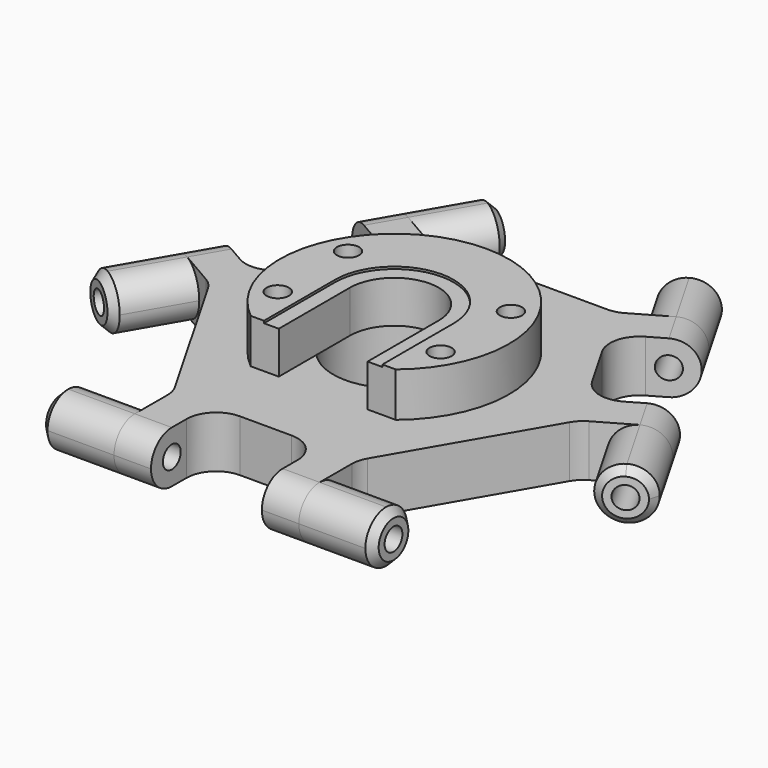
from build123d import *

# Parameters (mm, degrees)
F0_R      = 11
F0_R_2    = 8.25
F1_DEPTH  = 7
F2_W      = 5
F2_H      = 7
F3_DEPTH  = 10
F5_DEPTH  = 10
F6_R      = 1.5
F7_DEPTH  = 25
F8_SIZE   = 1
F10_DEPTH = 10
F11_R     = 1.5
F12_DEPTH = 25
F14_W     = 5
F14_H     = 7
F15_DEPTH = 10
F17_DEPTH = 10
F18_R     = 1.5
F19_DEPTH = 25
F20_SIZE  = 1
F22_DEPTH = 10
F23_R     = 1.5
F24_DEPTH = 25
F26_W     = 5
F26_H     = 7
F27_DEPTH = 10
F29_DEPTH = 10
F30_R     = 1.5
F31_DEPTH = 25
F32_SIZE  = 1
F34_DEPTH = 10
F35_R     = 1.5
F36_DEPTH = 25
F38_R     = 1.5
F39_DEPTH = 25
F40_R     = 3.4999
F41_R     = 4
F42_R     = 1.5
F43_DEPTH = 6
F45_DEPTH = 0.3
F46_R     = 10
F46_R_2   = 8.25
F47_DEPTH = 2


# Not quite as in the source:
# - a fillet or chamfer that OpenCascade refuses, or shapes differently, is made with other operations: its cross-section is extruded or revolved along the edge and cut away or added
# - a fillet or chamfer is up to 0.001 mm smaller than in the source, because OpenCascade refuses the exact size


with BuildPart() as f1:
    # F0 (on Top) → F1 (new body)
    with BuildSketch(Plane.XY):
        Polygon((24.999952403, -0.0487836684), (12.5422240976, 21.6262020402), (-12.4577283054, 21.6749857086), (-24.999952403, 0.0487836684), (-12.5422240976, -21.6262020402), (12.4577283054, -21.6749857086), align=None)
        Circle(F0_R, mode=Mode.SUBTRACT)
        Circle(F0_R)
        Circle(F0_R_2, mode=Mode.SUBTRACT)
    extrude(amount=F1_DEPTH)

    # F2 (on face) → F3 (join)
    with BuildSketch(Plane(origin=(-0.0422478961, -21.6505938744, 0), x_dir=(0.9999980961, -0.0019513467, 0), z_dir=(-0.0019513467, -0.9999980961, 0))):
        with Locations((-10, 3.5)):
            Rectangle(F2_W, F2_H)
        with Locations((10, 3.5)):
            Rectangle(F2_W, F2_H)
    extrude(amount=F3_DEPTH)

    # F4 (on face) → F5 (join)
    with BuildSketch(Plane(origin=(-12.4999762015, 0.0243918342, 0), x_dir=(-0.0019513467, -0.9999980961, 0), z_dir=(-0.9999980961, 0.0019513467, 0))):
        with BuildLine():
            ThreePointArc((28.1506350946, 0), (30.6255088288, 1.0251262658), (31.6506350946, 3.5))
            ThreePointArc((31.6506350946, 3.5), (30.6255088288, 5.9748737342), (28.1506350946, 7))
            ThreePointArc((28.1506350946, 7), (24.6506350946, 3.5), (28.1506350946, 0))
        make_face()
    extrude(amount=F5_DEPTH)

    # F6 (on face) → F7 (cut)
    with BuildSketch(Plane(origin=(-22.4999571627, 0.0439053016, 0), x_dir=(-0.0019513467, -0.9999980961, 0), z_dir=(-0.9999980961, 0.0019513467, 0))):
        with Locations((28.1506350946, 3.5)):
            Circle(F6_R)
    extrude(amount=-F7_DEPTH, mode=Mode.SUBTRACT)

    # F8
    f8_edges = [f1.edges().sort_by_distance(p)[0] for p in [
        (-22.554889, -28.106676, 7),
    ]]
    chamfer(f8_edges, length=F8_SIZE)

    # F9 (on face) → F10 (join)
    with BuildSketch(Plane(origin=(12.4999762015, -0.0243918342, 0), x_dir=(0.0019513467, 0.9999980961, 0), z_dir=(0.9999980961, -0.0019513467, 0))):
        with BuildLine():
            ThreePointArc((-28.1506350946, 0), (-25.6757613605, 1.0251262658), (-24.6506350946, 3.5))
            ThreePointArc((-24.6506350946, 3.5), (-25.6757613605, 5.9748737342), (-28.1506350946, 7))
            ThreePointArc((-28.1506350946, 7), (-30.6255088288, 5.9748737342), (-31.6506350946, 3.5))
            ThreePointArc((-31.6506350946, 3.5), (-30.6255088288, 1.0251262658), (-28.1506350946, 0))
        make_face()
    extrude(amount=F10_DEPTH)

    # F11 (on face) → F12 (cut)
    with BuildSketch(Plane(origin=(22.4999571627, -0.0439053016, 0), x_dir=(0.0019513467, 0.9999980961, 0), z_dir=(0.9999980961, -0.0019513467, 0))):
        with Locations((-28.1506350946, 3.5)):
            Circle(F11_R)
    extrude(amount=-F12_DEPTH, mode=Mode.SUBTRACT)

    # F13: chamfer of 1 on 1 edges, made by hand

    # F13_s1 → F13_t2 (revolve, cut)
    with BuildSketch(Plane.XY.offset(3.5)):
        Polygon((21.4381977031, -31.6925287905), (22.440147146, -30.6944820411), (22.4381957992, -31.6944801372), align=None)
    revolve(axis=Axis((22.4450255128, -28.1944868008, 3.5), (-0.9999980961, 0.0019513467, 0)), mode=Mode.SUBTRACT)

    # F14 (on face) → F15 (join)
    with BuildSketch(Plane(origin=(18.7710882503, 10.7887091859, 0), x_dir=(-0.4983091322, 0.8669994283, 0), z_dir=(0.8669994283, 0.4983091322, 0))):
        with Locations((-10, 3.5)):
            Rectangle(F14_W, F14_H)
        with Locations((10, 3.5)):
            Rectangle(F14_W, F14_H)
    extrude(amount=F15_DEPTH)

    # F16 (on face) → F17 (join)
    with BuildSketch(Plane(origin=(6.2288641527, -10.8374928543, 0), x_dir=(0.8669994283, 0.4983091322, 0), z_dir=(0.4983091322, -0.8669994283, 0))):
        with BuildLine():
            ThreePointArc((28.1506350946, 0), (30.6255088288, 1.0251262658), (31.6506350946, 3.5))
            ThreePointArc((31.6506350946, 3.5), (30.6255088288, 5.9748737342), (28.1506350946, 7))
            ThreePointArc((28.1506350946, 7), (24.6506350946, 3.5), (28.1506350946, 0))
        make_face()
    extrude(amount=F17_DEPTH)

    # F18 (on face) → F19 (cut)
    with BuildSketch(Plane(origin=(11.2119554749, -19.5074871378, 0), x_dir=(0.8669994283, 0.4983091322, 0), z_dir=(0.4983091322, -0.8669994283, 0))):
        with Locations((28.1506350946, 3.5)):
            Circle(F18_R)
    extrude(amount=-F19_DEPTH, mode=Mode.SUBTRACT)

    # F20
    f20_edges = [f1.edges().sort_by_distance(p)[0] for p in [
        (35.61854, -5.479769, 7),
    ]]
    chamfer(f20_edges, length=F20_SIZE)

    # F21 (on face) → F22 (join)
    with BuildSketch(Plane(origin=(-6.2288641527, 10.8374928543, 0), x_dir=(-0.8669994283, -0.4983091322, 0), z_dir=(-0.4983091322, 0.8669994283, 0))):
        with BuildLine():
            ThreePointArc((-28.1506350946, 0), (-25.6757613605, 1.0251262658), (-24.6506350946, 3.5))
            ThreePointArc((-24.6506350946, 3.5), (-25.6757613605, 5.9748737342), (-28.1506350946, 7))
            ThreePointArc((-28.1506350946, 7), (-30.6255088288, 5.9748737342), (-31.6506350946, 3.5))
            ThreePointArc((-31.6506350946, 3.5), (-30.6255088288, 1.0251262658), (-28.1506350946, 0))
        make_face()
    extrude(amount=F22_DEPTH)

    # F23 (on face) → F24 (cut)
    with BuildSketch(Plane(origin=(-11.2119554749, 19.5074871378, 0), x_dir=(-0.8669994283, -0.4983091322, 0), z_dir=(-0.4983091322, 0.8669994283, 0))):
        with Locations((-28.1506350946, 3.5)):
            Circle(F23_R)
    extrude(amount=-F24_DEPTH, mode=Mode.SUBTRACT)

    # F25: chamfer of 1 on 1 edges, made by hand

    # F25_s1 → F25_t2 (revolve, cut)
    with BuildSketch(Plane.XY.offset(3.5)):
        Polygon((16.7274361911, 34.4122882175), (15.3621276306, 34.7809785136), (16.2291270589, 35.2792876458), align=None)
    revolve(axis=Axis((13.1946290597, 33.5352056831, 3.5), (0.4983091322, -0.8669994283, 0)), mode=Mode.SUBTRACT)

    # F26 (on face) → F27 (join)
    with BuildSketch(Plane(origin=(-18.7288403542, 10.8618846885, 0), x_dir=(-0.5016889639, -0.8650480816, 0), z_dir=(-0.8650480816, 0.5016889639, 0))):
        with Locations((10, 3.5)):
            Rectangle(F26_W, F26_H)
        with Locations((-10, 3.5)):
            Rectangle(F26_W, F26_H)
    extrude(amount=F27_DEPTH)

    # F28 (on face) → F29 (join)
    with BuildSketch(Plane(origin=(6.2711120488, 10.8131010201, 0), x_dir=(-0.8650480816, 0.5016889639, 0), z_dir=(0.5016889639, 0.8650480816, 0))):
        with BuildLine():
            ThreePointArc((28.1506350946, 0), (30.6255088288, 1.0251262658), (31.6506350946, 3.5))
            ThreePointArc((31.6506350946, 3.5), (30.6255088288, 5.9748737342), (28.1506350946, 7))
            ThreePointArc((28.1506350946, 7), (24.6506350946, 3.5), (28.1506350946, 0))
        make_face()
    extrude(amount=F29_DEPTH)

    # F30 (on face) → F31 (cut)
    with BuildSketch(Plane(origin=(11.2880016879, 19.4635818362, 0), x_dir=(-0.8650480816, 0.5016889639, 0), z_dir=(0.5016889639, 0.8650480816, 0))):
        with Locations((28.1506350946, 3.5)):
            Circle(F30_R)
    extrude(amount=-F31_DEPTH, mode=Mode.SUBTRACT)

    # F32
    f32_edges = [f1.edges().sort_by_distance(p)[0] for p in [
        (-13.063651, 33.586445, 7),
    ]]
    chamfer(f32_edges, length=F32_SIZE)

    # F33 (on face) → F34 (join)
    with BuildSketch(Plane(origin=(-6.2711120488, -10.8131010201, 0), x_dir=(0.8650480816, -0.5016889639, 0), z_dir=(-0.5016889639, -0.8650480816, 0))):
        with BuildLine():
            ThreePointArc((-28.1506350946, 0), (-25.6757613605, 1.0251262658), (-24.6506350946, 3.5))
            ThreePointArc((-24.6506350946, 3.5), (-25.6757613605, 5.9748737342), (-28.1506350946, 7))
            ThreePointArc((-28.1506350946, 7), (-30.6255088288, 5.9748737342), (-31.6506350946, 3.5))
            ThreePointArc((-31.6506350946, 3.5), (-30.6255088288, 1.0251262658), (-28.1506350946, 0))
        make_face()
    extrude(amount=F34_DEPTH)

    # F35 (on face) → F36 (cut)
    with BuildSketch(Plane(origin=(-11.2880016879, -19.4635818362, 0), x_dir=(0.8650480816, -0.5016889639, 0), z_dir=(-0.5016889639, -0.8650480816, 0))):
        with Locations((-28.1506350946, 3.5)):
            Circle(F35_R)
    extrude(amount=-F36_DEPTH, mode=Mode.SUBTRACT)

    # F37: chamfer of 1 on 1 edges, made by hand

    # F37_s1 → F37_t2 (revolve, cut)
    with BuildSketch(Plane.XY.offset(3.5)):
        Polygon((-38.1656338943, -2.719759427), (-37.8022747766, -4.0864964725), (-38.6673228582, -3.5848075086), align=None)
    revolve(axis=Axis((-35.6396545725, -5.3407188823, 3.5), (0.5016889639, 0.8650480816, 0)), mode=Mode.SUBTRACT)

    # F38 (on face) → F39 (cut)
    with BuildSketch(Plane.XY.offset(7)):
        with Locations((-11, 5.9371710435)):
            Circle(F38_R)
        with Locations((11, 5.9371710435)):
            Circle(F38_R)
        with Locations((11, -5.9371710435)):
            Circle(F38_R)
        with Locations((-11, -5.9371710435)):
            Circle(F38_R)
    extrude(amount=-F39_DEPTH, mode=Mode.SUBTRACT)

    # F40 (radius 3.5 in the source; OpenCascade refuses exactly that, so slightly less here)
    f40_edges = [f1.edges().sort_by_distance(p)[0] for p in [
        (-10.061742, -31.631061, 7),
        (-10.061742, -31.631061, 0),
        (9.93822, -31.670088, 0),
        (9.93822, -31.670088, 7),
        (32.424174, 7.101806, 0),
        (32.424174, 7.101806, 7),
        (22.457991, 24.441795, 0),
        (22.457991, 24.441795, 7),
        (-22.362432, 24.529255, 0),
        (-22.362432, 24.529255, 7),
        (-32.396211, 7.228294, 0),
        (-32.396211, 7.228294, 7),
    ]]
    fillet(f40_edges, radius=F40_R)

    # F41
    f41_edges = [f1.edges().sort_by_distance(p)[0] for p in [
        (-24.999952, 0.048784, 3.5),
        (-12.542224, -21.626202, 3.5),
        (7.457738, -21.665229, 3.5),
        (-7.542234, -21.635959, 3.5),
        (12.457728, -21.674986, 3.5),
        (24.999952, -0.048784, 3.5),
        (22.508407, 4.286213, 3.5),
        (15.03377, 17.291205, 3.5),
        (12.542224, 21.626202, 3.5),
        (-12.457728, 21.674986, 3.5),
        (-14.966173, 17.349745, 3.5),
        (-22.491508, 4.374024, 3.5),
    ]]
    fillet(f41_edges, radius=F41_R)

    # F46 (on face) → F47 (join)
    with BuildSketch(Plane(origin=(0, 0, 0), x_dir=(1, 0, 0), z_dir=(0, 0, -1))):
        Circle(F46_R)
        Circle(F46_R_2, mode=Mode.SUBTRACT)
    extrude(amount=F47_DEPTH)


with BuildPart() as f43:
    # F42 (on face) → F43 (new body)
    with BuildSketch(Plane.XY.offset(7)):
        with BuildLine():
            ThreePointArc((-6, 0), (0, 6), (6, 0))
            Line((6, 0), (6, -5.6623758265))
            ThreePointArc((6, -5.6623758265), (7.6668931126, -3.0465144017), (8.25, 0))
            ThreePointArc((8.25, 0), (-3.0465144017, 7.6668931126), (-6, -5.6623758265))
            Line((-6, -5.6623758265), (-6, 0))
        make_face()
        with BuildLine():
            ThreePointArc((8.25, 0), (7.6668931126, -3.0465144017), (6, -5.6623758265))
            Line((6, -5.6623758265), (6, -12.0105544532))
            Line((6, -12.0105544532), (9.7977845316, -12.0105544532))
            ThreePointArc((9.7977845316, -12.0105544532), (0, 15.5), (-9.7977845316, -12.0105544532))
            Line((-9.7977845316, -12.0105544532), (-6, -12.0105544532))
            Line((-6, -12.0105544532), (-6, -5.6623758265))
            ThreePointArc((-6, -5.6623758265), (-3.0465144017, 7.6668931126), (8.25, 0))
        make_face()
        with Locations((-11, -5.9371710435)):
            Circle(F42_R, mode=Mode.SUBTRACT)
        with Locations((11, -5.9371710435)):
            Circle(F42_R, mode=Mode.SUBTRACT)
        with Locations((-11, 5.9371710435)):
            Circle(F42_R, mode=Mode.SUBTRACT)
        with Locations((11, 5.9371710435)):
            Circle(F42_R, mode=Mode.SUBTRACT)
    extrude(amount=F43_DEPTH)

    # F44 (on face) → F45 (cut)
    with BuildSketch(Plane.XY.offset(13)):
        with BuildLine():
            Line((8, -12.0105544532), (8, 0))
            ThreePointArc((8, 0), (0, 8), (-8, 0))
            Line((-8, 0), (-8, -12.0105544532))
            Line((-8, -12.0105544532), (-6, -12.0105544532))
            Line((-6, -12.0105544532), (-6, 0))
            ThreePointArc((-6, 0), (0, 6), (6, 0))
            Line((6, 0), (6, -12.0105544532))
            Line((6, -12.0105544532), (8, -12.0105544532))
        make_face()
    extrude(amount=-F45_DEPTH, mode=Mode.SUBTRACT)


solid = Compound([f1.part, f43.part])
